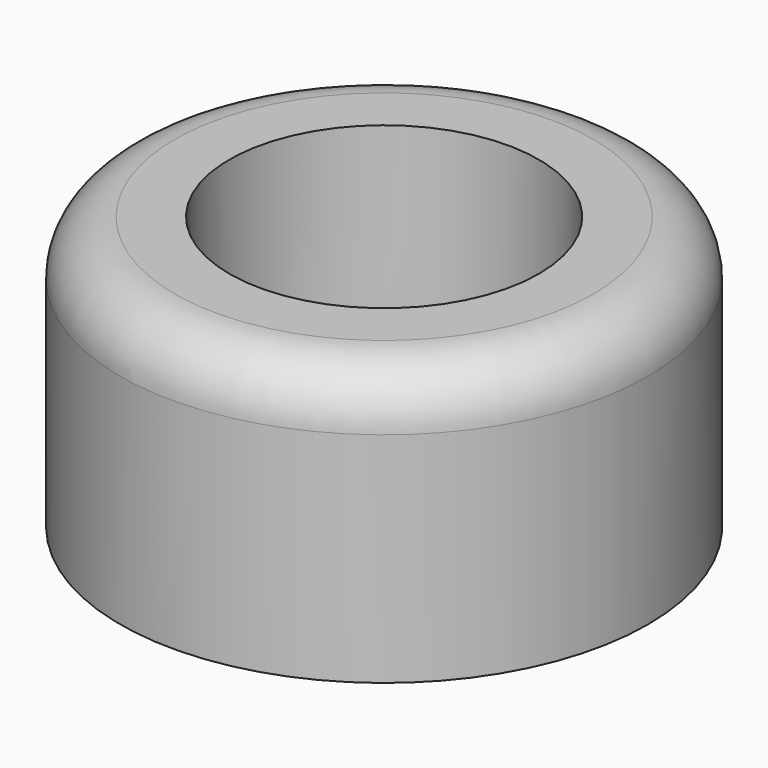
from build123d import *

# Parameters (mm, degrees)
F4_R     = 7.25
F4_R_2   = 4.25
F5_DEPTH = 7.5
F4_R_3   = 2.25
F6_DEPTH = 3
F7_R     = 1.5


# Not quite as in the source:
# - a feature of the source that left no trace in its solid (it failed there, or was rolled back) is left out


with BuildPart() as f5:
    # F4 (on Top) → F5 (new body)
    with BuildSketch(Plane.XY):
        Circle(F4_R)
        Circle(F4_R_2, mode=Mode.SUBTRACT)
    extrude(amount=F5_DEPTH)

    # F4 (on Top) → F6 (join)
    with BuildSketch(Plane.XY):
        Circle(F4_R_2)
        Circle(F4_R_3, mode=Mode.SUBTRACT)
    extrude(amount=F6_DEPTH)

    # F7
    f7_edges = [f5.edges().sort_by_distance(p)[0] for p in [
        (-7.25, 0, 7.5),
    ]]
    fillet(f7_edges, radius=F7_R)


solid = f5.part
